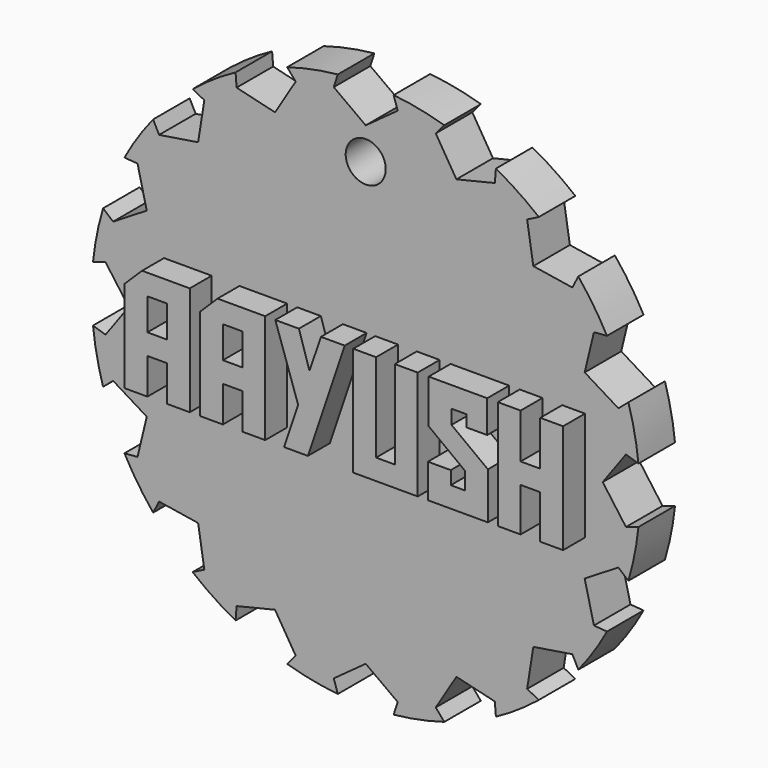
from build123d import *

# Parameters (mm, degrees)
F0_W            = 30.0037506968
F0_H            = 5.0006252714
F2_W            = 2.1300309692
F2_H            = 3.4757482194
F3_DEPTH        = 3
F5_DEPTH        = 25.4
F5_COPIES_COUNT = 16
F6_R            = 2.1907247283
F7_DEPTH        = 25.4


# Not quite as in the source:
# - a pattern or mirror of a feature is missing from the dataset's text; its kind, count and spacing are read off the source's solid


with BuildPart() as f1:
    # F0 (on Top) → F1 (revolve)
    with BuildSketch(Plane.XY):
        with Locations((-15.0018753484, 2.5003126357)):
            Rectangle(F0_W, F0_H)
    revolve(axis=Axis((0, 2.5003126357, 0), (0, 1, 0)))

    # F2 (on Front) → F3 (join)
    with BuildSketch(Plane.XZ):
        Polygon((-23.9999873, -5.969027547), (-21.4901833895, -5.969027547), (-21.4901833895, -2.0474589035), (-19.3601524204, -2.0474589035), (-19.3601524204, -5.969027547), (-16.8586044392, -5.969027547), (-16.8586044392, 5.969052947), (-22.0763547086, 5.969052947), (-23.9999873, 4.0784440727), align=None)
        with Locations((-20.425167905, 1.9607970218)):
            Rectangle(F2_W, F2_H, mode=Mode.SUBTRACT)
        Polygon((-15.7440533546, -5.969027547), (-13.2342494442, -5.969027547), (-13.2342494442, -2.0474589035), (-11.104218475, -2.0474589035), (-11.104218475, -5.969027547), (-8.6026704938, -5.969027547), (-8.6026704938, 5.969052947), (-13.8204207632, 5.969052947), (-15.7440533546, 4.0784440727), align=None)
        with Locations((-12.1692339596, 1.9607970218)):
            Rectangle(F2_W, F2_H, mode=Mode.SUBTRACT)
        Polygon((0.0990839243, 5.969052947), (-2.5015353055, 5.969052947), (-3.7564372364, 2.2703945398), (-4.912268016, 5.969052947), (-7.4963753385, 5.969052947), (-4.9948273574, -1.4034960795), (-6.5386870075, -5.969027547), (-3.9298118485, -5.969027547), align=None)
        Polygon((1.0320044675, -5.969027547), (8.0908279869, -5.969027547), (8.0908279869, 5.969052947), (5.5810240764, 5.969052947), (5.5810240764, -3.7069016607), (3.5335524487, -3.7069016607), (3.5335524487, 5.969052947), (1.0320044675, 5.969052947), align=None)
        Polygon((9.2053790715, -5.969027547), (15.7688465425, -5.969027547), (15.7688465425, -0.8586044554), (11.789486394, 2.1300436449), (11.789486394, 3.6904151536), (13.4241613148, 3.6904151536), (13.4241613148, 2.4190013641), (15.6945431303, 2.4190013641), (15.6945431303, 5.969052947), (9.2879384129, 5.969052947), (9.2879384129, 1.1888671724), (13.259042632, -1.8080368572), (13.259042632, -3.7069016607), (11.7069270526, -3.7069016607), (11.7069270526, -2.2538572813), (9.2053790715, -2.2538572813), align=None)
        Polygon((21.4984647188, 1.0650281846), (19.3519218911, 1.0650281846), (19.3519218911, 5.969052947), (16.8503739099, 5.969052947), (16.8503739099, -5.969027547), (19.3519218911, -5.969027547), (19.3519218911, -1.1970977017), (21.4984647188, -1.1970977017), (21.4984647188, -5.969027547), (24.0000127, -5.969027547), (24.0000127, 5.969052947), (21.4984647188, 5.969052947), align=None)
    extrude(amount=F3_DEPTH)

    # F4 (on Front) → F5 (cut)
    with BuildSketch(Plane.XZ):
        Polygon((2.1630311815, 32.5962975621), (-2.1630311815, 32.5962975621), (-3.4998579704, 28.4819677619), (0, 25.9391721044), (3.4998579704, 28.4819677619), align=None)
    f5 = extrude(amount=-F5_DEPTH, mode=Mode.SUBTRACT)

    # F5_copies: F5 ×16 about axis
    f5_copies_axis = Axis((0, 0, 0), (0, 1, 0))
    for i in range(1, F5_COPIES_COUNT):
        add(f5.rotate(f5_copies_axis, i * 360 / F5_COPIES_COUNT), mode=Mode.SUBTRACT)

    # F6 (on Front) → F7 (cut)
    with BuildSketch(Plane.XZ):
        with Locations((0, 22.427463904)):
            Circle(F6_R)
    extrude(amount=-F7_DEPTH, mode=Mode.SUBTRACT)


solid = f1.part
